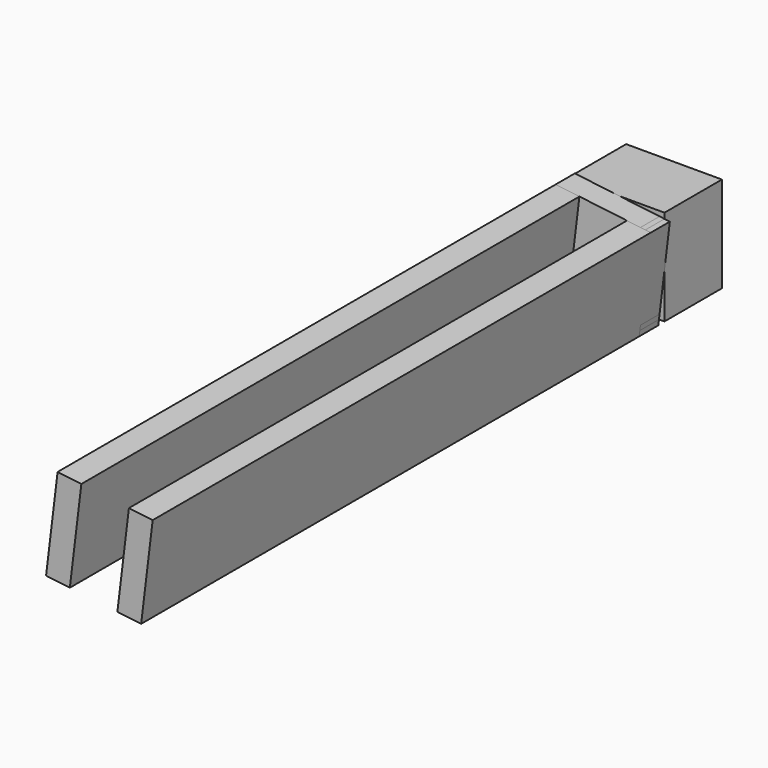
from build123d import *

# Parameters (mm, degrees)
F0_W     = 100
F0_H     = 100
F1_DEPTH = 75
F3_DEPTH = 25
F5_DEPTH = 650


# Not quite as in the source:
# - a feature names something its author has since deleted; it is built from what else it names


with BuildPart() as f1:
    # F0 (on Front) → F1 (new body)
    with BuildSketch(Plane.XZ):
        with Locations((50, 50)):
            Rectangle(F0_W, F0_H)
    extrude(amount=F1_DEPTH)

    # F2 (on face) → F3 (join)
    with BuildSketch(Plane.XZ.offset(75)):
        Polygon((100, 94.3057966884), (100, 46.974800806), (105.6538372319, 93.6205058254), align=None)
        Polygon((94.9213680166, 94.9213680166), (50, 50), (94.9217934551, 5.0782065449), (100, 46.974800806), (100, 94.3057966884), align=None)
        Polygon((0, 53.0131088143), (-5.6523319044, 6.3798231584), (0, 5.6947147534), align=None)
        Polygon((6.3804113302, 105.6532490601), (5.6951917585, 100), (53.0212637714, 100), align=None)
        Polygon((94.3062736934, 0), (46.9829557631, 0), (93.6210939972, -5.6529200762), align=None)
        Polygon((5.6951917585, 100), (5.0795135743, 94.9204864257), (50, 50), (94.9213680166, 94.9213680166), (53.0212637714, 100), align=None)
        Polygon((50, 50), (5.0790881358, 5.0790881358), (46.9829557631, 0), (94.3062736934, 0), (94.9217934551, 5.0782065449), align=None)
        Polygon((5.0795135743, 94.9204864257), (0, 53.0131088143), (0, 5.6947147534), (5.0790881358, 5.0790881358), (50, 50), align=None)
    extrude(amount=F3_DEPTH)

    # F4 (on face) → F5 (join)
    with BuildSketch(Plane.XZ.offset(100)):
        Polygon((31.1987678056, 102.6450632514), (6.3804113302, 105.6532490601), (-5.6523319044, 6.3798231584), (19.166024571, 3.3716373498), align=None)
        Polygon((93.6210939972, -5.6529200762), (105.6538372319, 93.6205058254), (80.8354807565, 96.6286916341), (68.8027375218, -2.6447342676), align=None)
    extrude(amount=F5_DEPTH)


solid = f1.part
